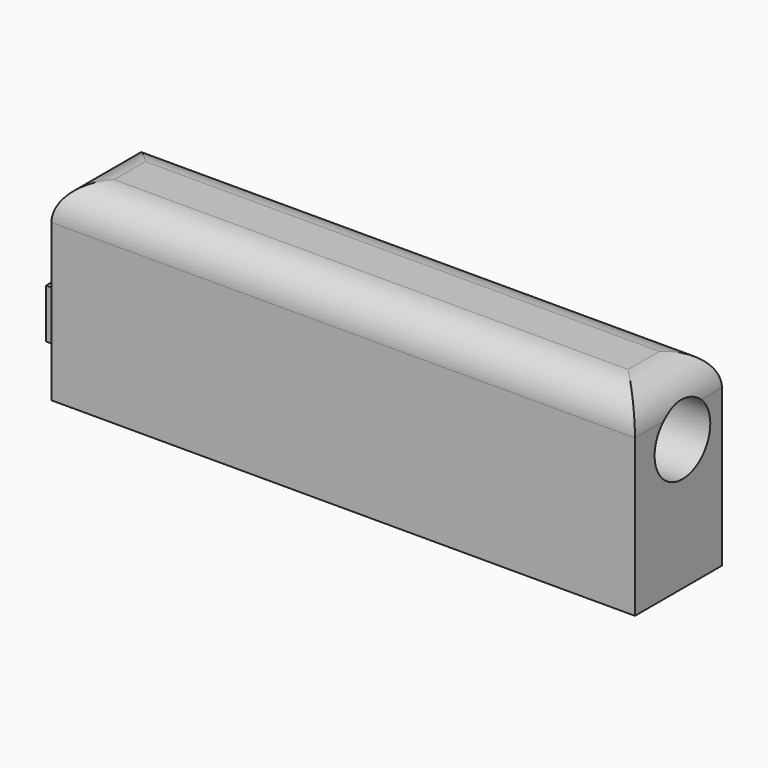
from build123d import *

# Parameters (mm, degrees)
F0_W        = 42.580999434
F0_H        = 7.9333577305
F1_DEPTH    = 13.97
F2_R        = 2.54
F3_DEPTH    = 45.0342
F4_T1_DEPTH = 20.6333577305
F4_T3_DEPTH = 55.280999434
F5_W        = 2.8782505542
F5_H        = 3.5978133092
F5_W_2      = 1.7989068292
F5_H_2      = 2.7433328796
F6_DEPTH    = 3.1496


# Not quite as in the source:
# - a fillet or chamfer that OpenCascade refuses, or shapes differently, is made with other operations: its cross-section is extruded or revolved along the edge and cut away or added


with BuildPart() as f1:
    # F0 (on Top) → F1 (new body)
    with BuildSketch(Plane.XY):
        with Locations((21.290499717, 3.9666788653)):
            Rectangle(F0_W, F0_H)
    extrude(amount=F1_DEPTH)

    # F2 (on Right) → F3 (cut)
    with BuildSketch(Plane.YZ):
        with Locations((4.3319589458, 9.5625361428)):
            Circle(F2_R)
    extrude(amount=F3_DEPTH, mode=Mode.SUBTRACT)

    # F4: fillet of radius 2.54 on 4 edges, made by hand

    # F4_s2 → F4_t1 (cut)
    with BuildSketch(Plane.XZ.offset(-14.2833577305)):
        with BuildLine():
            ThreePointArc((0, 11.43), (0.7439487758, 13.2260512242), (2.54, 13.97))
            Line((2.54, 13.97), (0, 13.97))
            Line((0, 13.97), (0, 11.43))
        make_face()
        with BuildLine():
            ThreePointArc((40.040999434, 13.97), (41.8370506582, 13.2260512242), (42.580999434, 11.43))
            Line((42.580999434, 11.43), (42.580999434, 13.97))
            Line((42.580999434, 13.97), (40.040999434, 13.97))
        make_face()
    extrude(amount=F4_T1_DEPTH, mode=Mode.SUBTRACT)

    # F4_s4 → F4_t3 (cut)
    with BuildSketch(Plane.YZ.offset(-6.35)):
        with BuildLine():
            ThreePointArc((7.9333577305, 11.43), (7.1894089547, 13.2260512242), (5.3933577305, 13.97))
            Line((5.3933577305, 13.97), (7.9333577305, 13.97))
            Line((7.9333577305, 13.97), (7.9333577305, 11.43))
        make_face()
        with BuildLine():
            ThreePointArc((2.54, 13.97), (0.7439487758, 13.2260512242), (0, 11.43))
            Line((0, 11.43), (0, 13.97))
            Line((0, 13.97), (2.54, 13.97))
        make_face()
    extrude(amount=F4_T3_DEPTH, mode=Mode.SUBTRACT)

    # F5 (on Right) → F6 (join)
    with BuildSketch(Plane.YZ):
        with Locations((4.8902533017, 3.1496292795)):
            Rectangle(F5_W, F5_H)
        with Locations((4.8902535345, 3.2170884078)):
            Rectangle(F5_W_2, F5_H_2, mode=Mode.SUBTRACT)
    extrude(amount=-F6_DEPTH)


solid = f1.part
